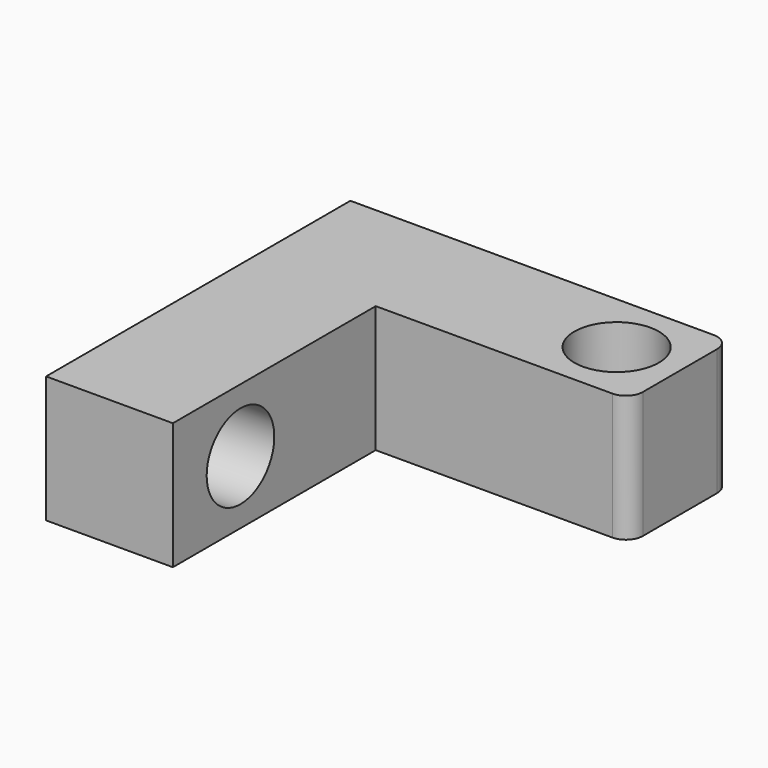
from build123d import *

# Parameters (mm, degrees)
F1_DEPTH = 19.05
F3_D     = 12.7
F4_R     = 2.54
F6_D     = 12.7


# Not quite as in the source:
# - a feature names something its author has since deleted; it is built from what else it names


with BuildPart() as f1:
    # F0 (on Top) → F1 (new body)
    with BuildSketch(Plane.XY):
        Polygon((-12.7313164792, 44.4748119943), (-12.7313164792, -12.6751880057), (6.3186835208, -12.6751880057), (6.3186835208, 25.4248119943), (44.4186835208, 25.4248119943), (44.4186835208, 44.4748119943), align=None)
    extrude(amount=F1_DEPTH)

    # F3 (through all)
    with Locations(Plane.XY.offset(19.05)):
        with Locations((34.8936835208, 34.9498119943)):
            Hole(F3_D / 2)

    # F4
    f4_edges = [f1.edges().sort_by_distance(p)[0] for p in [
        (44.418684, 25.424812, 9.525),
        (44.418684, 44.474812, 9.525),
    ]]
    fillet(f4_edges, radius=F4_R)

    # F6 (through all)
    with Locations(Plane.YZ.offset(6.3186835208)):
        with Locations((0.0248119943, 9.525)):
            Hole(F6_D / 2)


solid = f1.part
